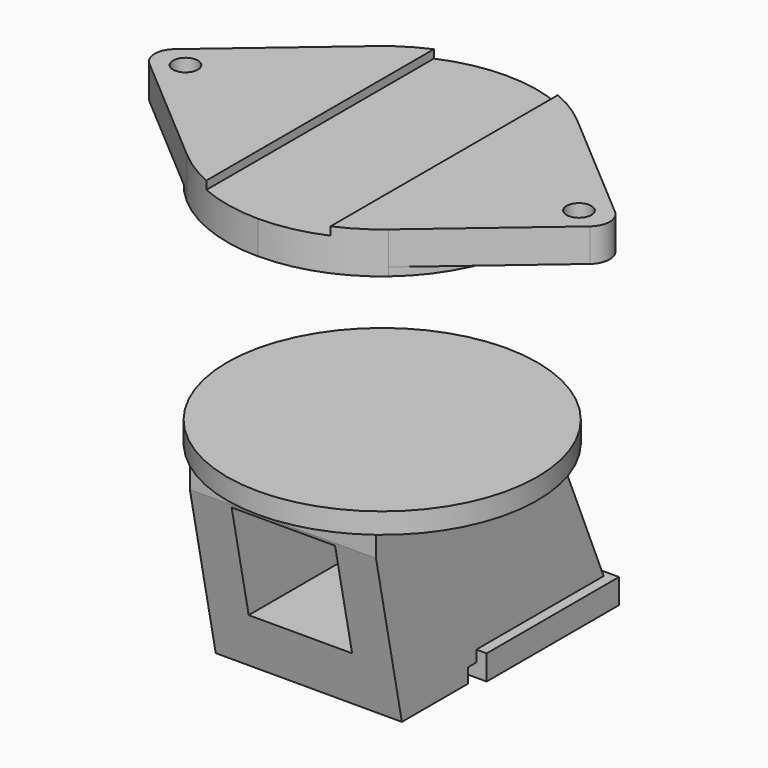
from build123d import *

# Parameters (mm, degrees)
F1_DEPTH  = 16
F2_DEPTH  = 20
F3_R      = 6
F4_DEPTH  = 16
F5_W      = 30
F5_H      = 4
F6_DEPTH  = 75
F8_R      = 75
F9_DEPTH  = 10
F12_DEPTH = 60
F13_DEPTH = 77.8
F15_DEPTH = 100
F16_W     = 77.1548634648
F16_H     = 3
F17_DEPTH = 45
F19_DEPTH = 50
F20_W     = 25
F20_H     = 50
F21_DEPTH = 80
F22_DEPTH = 80


with BuildPart() as f1:
    # F0 (on Top) → F1 (new body)
    with BuildSketch(Plane.XY):
        with BuildLine():
            ThreePointArc((-48.751355202, -56.9939063933), (-75, 0), (-48.751355202, 56.9939063933))
            Line((-48.751355202, 56.9939063933), (-106.4974008694, 7.5991875191))
            ThreePointArc((-106.4974008694, 7.5991875191), (-109.9972201758, 0), (-106.4974008694, -7.5991875191))
            Line((-106.4974008694, -7.5991875191), (-48.751355202, -56.9939063933))
        make_face()
    extrude(amount=-F1_DEPTH)

    # F0 (on Top) → F2 (join)
    with BuildSketch(Plane.XY):
        with BuildLine():
            Line((0, -75), (0, 75))
            ThreePointArc((0, 75), (-25.9851594232, 70.354612427), (-48.751355202, 56.9939063933))
            ThreePointArc((-48.751355202, 56.9939063933), (-75, 0), (-48.751355202, -56.9939063933))
            ThreePointArc((-48.751355202, -56.9939063933), (-25.9851594232, -70.354612427), (0, -75))
        make_face()
    extrude(amount=-F2_DEPTH)

    # F3 (on face) → F4 (cut)
    with BuildSketch(Plane(origin=(0, 0, -16), x_dir=(1, 0, 0), z_dir=(0, 0, -1))):
        with Locations((-95.1382219791, 0)):
            Circle(F3_R)
    extrude(amount=-F4_DEPTH, mode=Mode.SUBTRACT)

    # F5 (on Front) → F6 (cut, symmetric)
    with BuildSketch(Plane.XZ):
        with Locations((-15, -2)):
            Rectangle(F5_W, F5_H)
    extrude(amount=F6_DEPTH, both=True, mode=Mode.SUBTRACT)

    # F7: F1 across face


with BuildPart() as f1_1:
    add(f1.part)
    add(f1.part.mirror(Plane(origin=(0, 0, -12), x_dir=(0, 1, 0), z_dir=(1, 0, 0))))


with BuildPart() as f9:
    # F8 (on face) → F9 (new body)
    with BuildSketch(Plane(origin=(0, 0, -20), x_dir=(1, 0, 0), z_dir=(0, 0, -1))):
        Circle(F8_R)
    extrude(amount=F9_DEPTH)


with BuildPart() as f9_1:
    # F10: moved
    add(f9.part.moved(Location((0, 0, -100))))

    # F11 (on Front) → F12 (join)
    with BuildSketch(Plane.XZ):
        Polygon((0, -126), (-45, -126), (-45, -216), (45, -216), (45, -126), align=None)
    extrude(amount=F12_DEPTH)

    # F13 (add): a face of the model
    f13_faces = [f9_1.faces().sort_by_distance(p)[0] for p in [
        (0, 0, -173),
    ]]
    extrude(f13_faces, amount=F13_DEPTH)

    # F14 (on face) → F15 (cut)
    with BuildSketch(Plane.XY.offset(-120)):
        with BuildLine():
            ThreePointArc((75, 0), (53.033008589, -53.033008589), (0, -75))
            Line((0, -75), (93.311317265, -75))
            Line((93.311317265, -75), (93.311317265, 95.2438786626))
            Line((93.311317265, 95.2438786626), (0, 95.2438786626))
            Line((0, 95.2438786626), (0, 75))
            ThreePointArc((0, 75), (53.033008589, 53.033008589), (75, 0))
        make_face()
        with BuildLine():
            Line((0, 75), (0, -75))
            ThreePointArc((0, -75), (53.033008589, -53.033008589), (75, 0))
            ThreePointArc((75, 0), (53.033008589, 53.033008589), (0, 75))
        make_face()
    extrude(amount=-F15_DEPTH, mode=Mode.SUBTRACT)

    # F16 (on face) → F17 (cut)
    with BuildSketch(Plane(origin=(-45, 0, 0), x_dir=(0, -1, 0), z_dir=(-1, 0, 0))):
        Polygon((-77.8, -130), (-77.8, -204), (-53.6902993917, -146.880954504), (-53.6902993917, -130), align=None)
        with Locations((-39.2225682676, -214.5)):
            Rectangle(F16_W, F16_H)
        Polygon((60, -216), (60, -140), (44.3548634648, -216), align=None)
        Polygon((-0.6451365352, -216), (4.3548634648, -216), (4.3548634648, -213), (4.3548634648, -209), (-0.6451365352, -209), (-0.6451365352, -213), align=None)
    extrude(amount=-F17_DEPTH, mode=Mode.SUBTRACT)

    # F18 (on face) → F19 (join)
    with BuildSketch(Plane.YZ):
        Polygon((80.6451365352, -203.4836058617), (77.8, -203.4836058617), (77.5820322808, -203.4836058617), (77.8, -204), (77.8, -213), (0.6451365352, -213), (0.6451365352, -215.4836058617), (80.6451365352, -215.4836058617), align=None)
        Polygon((77.8, -204), (77.5820322808, -203.4836058617), (0.6451365352, -203.4836058617), (0.6451365352, -209), (0.6451365352, -213), (77.8, -213), align=None)
    extrude(amount=-F19_DEPTH)

    # F20 (on Front) → F21 (cut)
    with BuildSketch(Plane.XZ):
        with Locations((-12.5, -166.2339031696)):
            Rectangle(F20_W, F20_H)
    extrude(amount=-F21_DEPTH, mode=Mode.SUBTRACT)

    # F22 (cut): a face of the model
    f22_faces = [f9_1.faces().sort_by_distance(p)[0] for p in [
        (-12.5, 0, -166.2339031696),
    ]]
    extrude(f22_faces, amount=-F22_DEPTH, mode=Mode.SUBTRACT)

    # F23: F9 across face


with BuildPart() as f9_2:
    add(f9_1.part)
    add(f9_1.part.mirror(Plane(origin=(0, 15.3582634866, -203.4262275083), x_dir=(0, 1, 0), z_dir=(1, 0, 0))))


solid = Compound([f1_1.part, f9_2.part])
